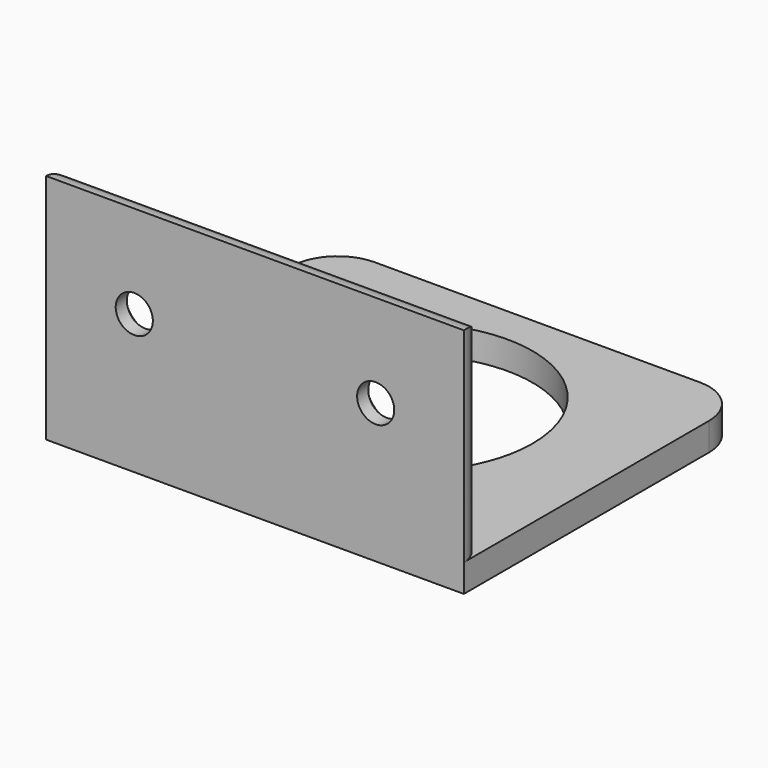
from build123d import *

# Parameters (mm, degrees)
F1_DEPTH       = 3
F0_W           = 45
F0_H           = 3
F2_DEPTH       = 25
F4_D           = 4
F4_CSINK_D     = 7
F4_CSINK_ANGLE = 90
F5_R           = 2.99999


# Not quite as in the source:
# - a fillet or chamfer is up to 0.001 mm smaller than in the source, because OpenCascade refuses the exact size


with BuildPart() as f1:
    # F0 (on Top) → F1 (new body)
    with BuildSketch(Plane.XY):
        with BuildLine():
            Line((0, 33), (0, 3))
            Line((0, 3), (45, 3))
            Line((45, 3), (45, 33))
            ThreePointArc((45, 33), (43.5355339059, 36.5355339059), (40, 38))
            Line((40, 38), (5, 38))
            ThreePointArc((5, 38), (1.4644660941, 36.5355339059), (0, 33))
        make_face()
        with BuildLine():
            add(Edge.make_bspline(
                [(36, 20.5), (36, 43.8826859022), (15.75, 32.1913429511), (-4.5, 20.5), (15.75, 8.8086570489), (36, -2.8826859022), (36, 20.5)],
                knots=[0, 0, 0, 2.0943951024, 2.0943951024, 4.1887902048, 4.1887902048, 6.2831853072, 6.2831853072, 6.2831853072], degree=2, weights=[1, 0.5, 1, 0.5, 1, 0.5, 1]))
        make_face(mode=Mode.SUBTRACT)
    extrude(amount=F1_DEPTH)

    # F0 (on Top) → F2 (join)
    with BuildSketch(Plane.XY):
        with Locations((22.5, 1.5)):
            Rectangle(F0_W, F0_H)
    extrude(amount=F2_DEPTH)

    # F4 (through all)
    with Locations(Plane(origin=(0, 3, 0), x_dir=(-1, 0, 0), z_dir=(0, 1, 0))):
        with Locations((-35.5, 15), (-9.5, 15)):
            CounterSinkHole(F4_D / 2, F4_CSINK_D / 2, counter_sink_angle=F4_CSINK_ANGLE)

    # F5 (radius 3 in the source; OpenCascade refuses exactly that, so slightly less here)
    f5_edges = [f1.edges().sort_by_distance(p)[0] for p in [
        (45, 3, 14),
        (22.5, 3, 25),
        (0, 3, 14),
    ]]
    fillet(f5_edges, radius=F5_R)


solid = f1.part
